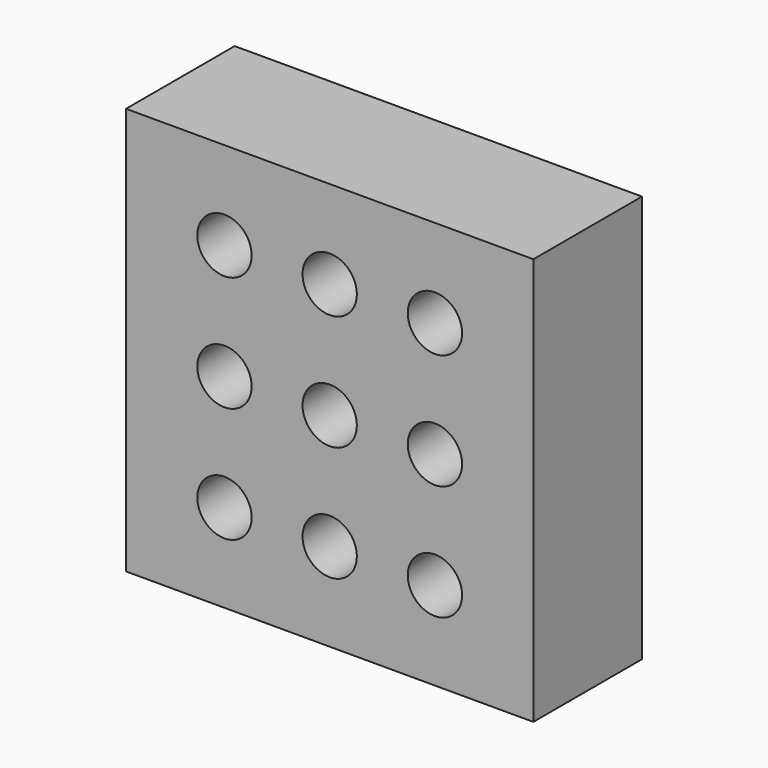
from build123d import *

# Parameters (mm, degrees)
F0_W         = 76.2
F0_H         = 76.2
F1_DEPTH     = 25.4
F2_R         = 5.08
F4_DEPTH     = 12.7
F3_TEXT_SIZE = 10.8738061196
F5_DEPTH     = 5.08


# Not quite as in the source:
# - Text() gives the source's letters only with a copy of the font that has no kerning and outlines rounded to 1/6400 em; it was checked with that copy


with BuildPart() as f1:
    # F0 (on Front) → F1 (new body)
    with BuildSketch(Plane.XZ):
        with Locations((38.1, 38.1)):
            Rectangle(F0_W, F0_H)
    extrude(amount=F1_DEPTH)

    # F2 (on face) → F4 (cut)
    with BuildSketch(Plane.XZ.offset(25.4)):
        with Locations((18.415, 59.69)):
            Circle(F2_R)
        with Locations((18.415, 38.1)):
            Circle(F2_R)
        with Locations((18.415, 16.51)):
            Circle(F2_R)
        with Locations((38.1, 59.69)):
            Circle(F2_R)
        with Locations((38.1, 38.1)):
            Circle(F2_R)
        with Locations((38.1, 16.51)):
            Circle(F2_R)
        with Locations((57.785, 59.69)):
            Circle(F2_R)
        with Locations((57.785, 38.1)):
            Circle(F2_R)
        with Locations((57.785, 16.51)):
            Circle(F2_R)
    extrude(amount=-F4_DEPTH, mode=Mode.SUBTRACT)

    # F3 (on face) → F5 (cut)
    with BuildSketch(Plane(origin=(0, 0, 0), x_dir=(1, 0, 0), z_dir=(0, 0, -1))):
        with Locations((7.7336635441, 8.4974826314)):
            Text("Mc.Donald's", F3_TEXT_SIZE, font='Open Sans', text_align=(TextAlign.LEFT, TextAlign.BOTTOM))
    extrude(amount=-F5_DEPTH, mode=Mode.SUBTRACT)


solid = f1.part
